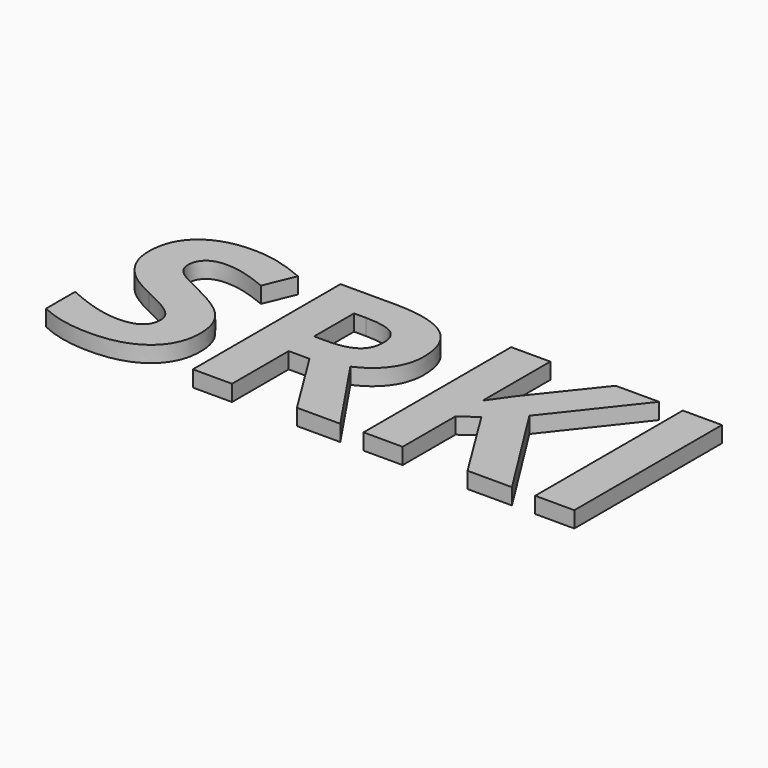
from build123d import *

# Parameters (mm, degrees)
F0_TEXT_SIZE = 32.0939895408
F1_DEPTH     = 2


# Not quite as in the source:
# - Text() gives the source's letters only with a copy of the font that has no kerning and outlines rounded to 1/6400 em; it was checked with that copy


with BuildPart() as f1:
    # F0 (on Top) → F1 (new body)
    with BuildSketch(Plane.XY):
        with Locations((-34.865417529, -9.8512022605)):
            Text('SRKI', F0_TEXT_SIZE, font='Open Sans', font_style=FontStyle.BOLD, text_align=(TextAlign.LEFT, TextAlign.BOTTOM))
    extrude(amount=F1_DEPTH)


solid = f1.part
